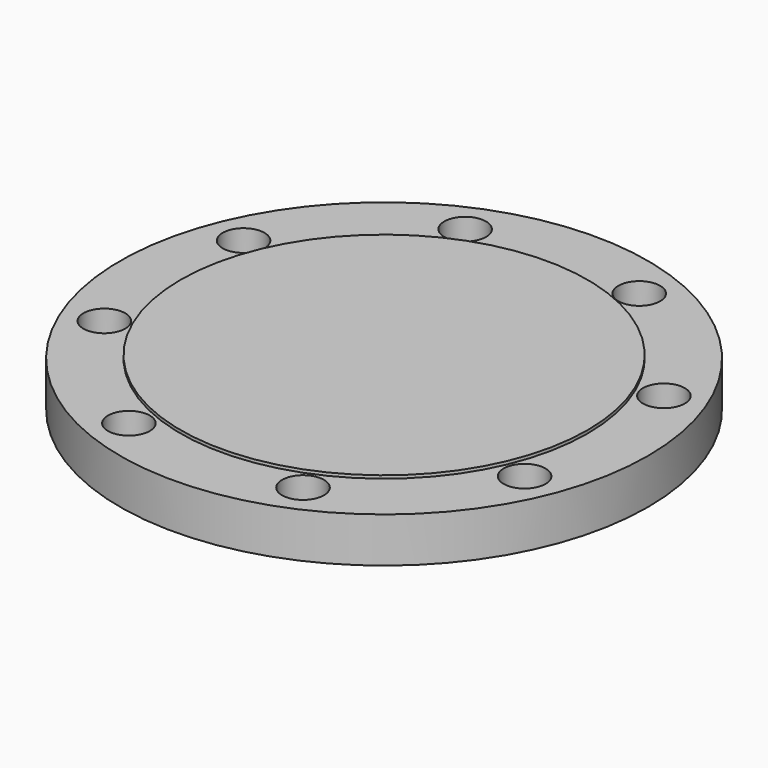
from build123d import *

# Parameters (mm, degrees)
F2_R     = 140
F2_R_2   = 11.1
F2_R_3   = 107.95
F4_DEPTH = 23.9
F5_DEPTH = 25.5


# Not quite as in the source:
# - a feature names something its author has since deleted; it is built from what else it names


with BuildPart() as f4:
    # F2 (on Top) → F4 (new body)
    with BuildSketch(Plane.XY):
        Circle(F2_R)
        with Locations((-46.1707561148, -111.4660655975)):
            Circle(F2_R_2, mode=Mode.SUBTRACT)
        with Locations((-111.4660655975, -46.1707561148)):
            Circle(F2_R_2, mode=Mode.SUBTRACT)
        with Locations((46.1707561148, -111.4660655975)):
            Circle(F2_R_2, mode=Mode.SUBTRACT)
        with Locations((111.4660655975, -46.1707561148)):
            Circle(F2_R_2, mode=Mode.SUBTRACT)
        with Locations((-111.4660655975, 46.1707561148)):
            Circle(F2_R_2, mode=Mode.SUBTRACT)
        with Locations((-46.1707561148, 111.4660655975)):
            Circle(F2_R_2, mode=Mode.SUBTRACT)
        Circle(F2_R_3, mode=Mode.SUBTRACT)
        with Locations((111.4660655975, 46.1707561148)):
            Circle(F2_R_2, mode=Mode.SUBTRACT)
        with Locations((46.1707561148, 111.4660655975)):
            Circle(F2_R_2, mode=Mode.SUBTRACT)
        Circle(F2_R_3)
    extrude(amount=F4_DEPTH)

    # F2 (on Top) → F5 (join)
    with BuildSketch(Plane.XY):
        Circle(F2_R_3)
    extrude(amount=F5_DEPTH)


solid = f4.part
